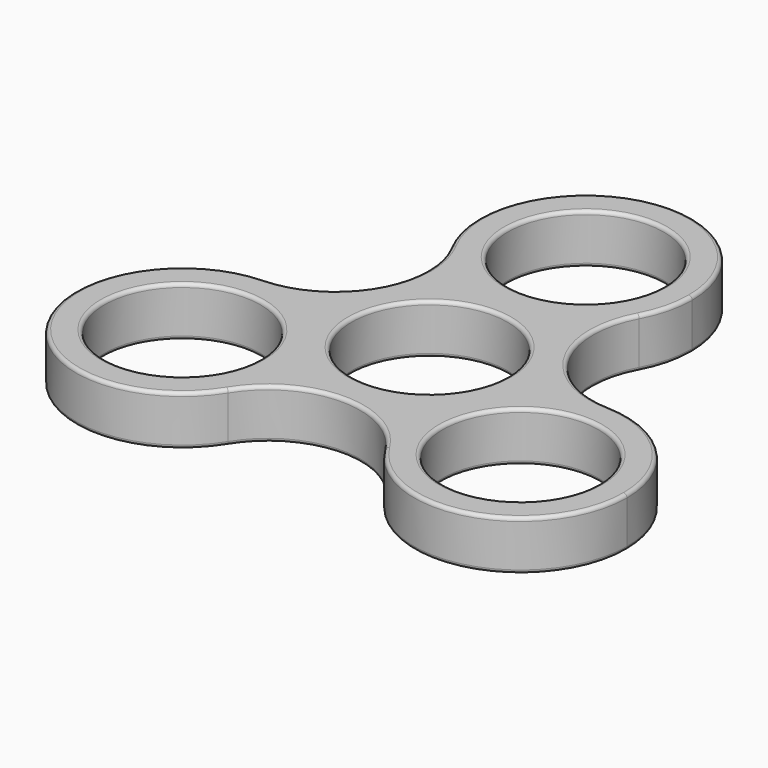
from build123d import *

# Parameters (mm, degrees)
F0_R     = 11
F1_DEPTH = 7
F2_R     = 0.5


# Not quite as in the source:
# - a feature names something its author has since deleted; it is built from what else it names


with BuildPart() as f1:
    # F0 (on Top) → F1 (new body)
    with BuildSketch(Plane.XY):
        with BuildLine():
            ThreePointArc((-61.119560109, 18.0493719403), (-59.7843480604, 21.4909475398), (-59.330106933, 25.1544020325))
            ThreePointArc((-59.330106933, 25.1544020325), (-77.9935614257, 39.7001609051), (-87.540653757, 18.0493719403))
            ThreePointArc((-87.540653757, 18.0493719403), (-84.4913145964, 14.1203701845), (-80.3248963371, 11.4044020325))
            ThreePointArc((-80.3248963371, 11.4044020325), (-74.330106933, 12.6544020325), (-68.3353175289, 11.4044020325))
            ThreePointArc((-68.3353175289, 11.4044020325), (-64.1688992696, 14.1203701845), (-61.119560109, 18.0493719403))
        make_face()
        with Locations((-74.330106933, 25.1544020325)):
            Circle(F0_R, mode=Mode.SUBTRACT)
        with BuildLine():
            ThreePointArc((-80.3248963371, 11.4044020325), (-84.4913145964, 14.1203701845), (-87.540653757, 18.0493719403))
            ThreePointArc((-87.540653757, 18.0493719403), (-87.7314640886, 5.3916791938), (-98.5979423946, -1.102413774))
            ThreePointArc((-98.5979423946, -1.102413774), (-93.6706574823, -1.7787180739), (-89.2353509371, -4.0289580532))
            ThreePointArc((-89.2353509371, -4.0289580532), (-87.3204879898, 5.1544020325), (-80.3248963371, 11.4044020325))
        make_face()
        with BuildLine():
            ThreePointArc((-50.0622714714, -1.102413774), (-60.9287497774, 5.3916791938), (-61.119560109, 18.0493719403))
            ThreePointArc((-61.119560109, 18.0493719403), (-64.1688992696, 14.1203701845), (-68.3353175289, 11.4044020325))
            ThreePointArc((-68.3353175289, 11.4044020325), (-61.7817635949, 5.8726183517), (-59.330106933, -2.3455979675))
            ThreePointArc((-59.330106933, -2.3455979675), (-59.3538146672, -3.1886104047), (-59.4248629289, -4.0289580532))
            ThreePointArc((-59.4248629289, -4.0289580532), (-54.9895563837, -1.7787180739), (-50.0622714714, -1.102413774))
        make_face()
        with BuildLine():
            ThreePointArc((-68.3353175289, 11.4044020325), (-74.330106933, 12.6544020325), (-80.3248963371, 11.4044020325))
            ThreePointArc((-80.3248963371, 11.4044020325), (-74.330106933, 10.1544020325), (-68.3353175289, 11.4044020325))
        make_face()
        with BuildLine():
            ThreePointArc((-68.3353175289, 11.4044020325), (-74.330106933, 10.1544020325), (-80.3248963371, 11.4044020325))
            ThreePointArc((-80.3248963371, 11.4044020325), (-87.3204879898, 5.1544020325), (-89.2353509371, -4.0289580532))
            ThreePointArc((-89.2353509371, -4.0289580532), (-85.1554244803, -8.5955979675), (-83.240561533, -14.4122378818))
            ThreePointArc((-83.240561533, -14.4122378818), (-74.330106933, -17.3455979675), (-65.419652333, -14.4122378818))
            ThreePointArc((-65.419652333, -14.4122378818), (-63.5047893857, -8.5955979675), (-59.4248629289, -4.0289580532))
            ThreePointArc((-59.4248629289, -4.0289580532), (-59.3538146672, -3.1886104047), (-59.330106933, -2.3455979675))
            ThreePointArc((-59.330106933, -2.3455979675), (-61.7817635949, 5.8726183517), (-68.3353175289, 11.4044020325))
        make_face()
        with Locations((-74.330106933, -2.3455979675)):
            Circle(F0_R, mode=Mode.SUBTRACT)
        with BuildLine():
            ThreePointArc((-89.2353509371, -4.0289580532), (-93.6706574823, -1.7787180739), (-98.5979423946, -1.102413774))
            ThreePointArc((-98.5979423946, -1.102413774), (-111.1361865938, -23.5955979675), (-85.3873955706, -23.9837520689))
            ThreePointArc((-85.3873955706, -23.9837520689), (-83.7170815897, -20.1958327476), (-83.1458055371, -16.0955979675))
            ThreePointArc((-83.1458055371, -16.0955979675), (-83.1695132713, -15.2525855304), (-83.240561533, -14.4122378818))
            ThreePointArc((-83.240561533, -14.4122378818), (-87.3204879898, -9.8455979675), (-89.2353509371, -4.0289580532))
        make_face()
        with Locations((-98.1458055371, -16.0955979675)):
            Circle(F0_R, mode=Mode.SUBTRACT)
        with BuildLine():
            ThreePointArc((-35.5144083289, -16.0955979675), (-39.7491388743, -5.650073875), (-50.0622714714, -1.102413774))
            ThreePointArc((-50.0622714714, -1.102413774), (-54.9895563837, -1.7787180739), (-59.4248629289, -4.0289580532))
            ThreePointArc((-59.4248629289, -4.0289580532), (-61.3397258762, -9.8455979675), (-65.419652333, -14.4122378818))
            ThreePointArc((-65.419652333, -14.4122378818), (-65.1507640471, -19.3784460131), (-63.2728182954, -23.9837520689))
            ThreePointArc((-63.2728182954, -23.9837520689), (-46.4141735489, -30.5243219149), (-35.5144083289, -16.0955979675))
        make_face()
        with Locations((-50.5144083289, -16.0955979675)):
            Circle(F0_R, mode=Mode.SUBTRACT)
        with BuildLine():
            ThreePointArc((-83.240561533, -14.4122378818), (-85.1554244803, -8.5955979675), (-89.2353509371, -4.0289580532))
            ThreePointArc((-89.2353509371, -4.0289580532), (-87.3204879898, -9.8455979675), (-83.240561533, -14.4122378818))
        make_face()
        with BuildLine():
            ThreePointArc((-83.1458055371, -16.0955979675), (-83.7170815897, -20.1958327476), (-85.3873955706, -23.9837520689))
            ThreePointArc((-85.3873955706, -23.9837520689), (-74.330106933, -17.8201522901), (-63.2728182954, -23.9837520689))
            ThreePointArc((-63.2728182954, -23.9837520689), (-65.1507640471, -19.3784460131), (-65.419652333, -14.4122378818))
            ThreePointArc((-65.419652333, -14.4122378818), (-74.330106933, -17.3455979675), (-83.240561533, -14.4122378818))
            ThreePointArc((-83.240561533, -14.4122378818), (-83.1695132713, -15.2525855304), (-83.1458055371, -16.0955979675))
        make_face()
        with BuildLine():
            ThreePointArc((-65.419652333, -14.4122378818), (-61.3397258762, -9.8455979675), (-59.4248629289, -4.0289580532))
            ThreePointArc((-59.4248629289, -4.0289580532), (-63.5047893857, -8.5955979675), (-65.419652333, -14.4122378818))
        make_face()
    extrude(amount=F1_DEPTH)

    # F2
    f2_edges = [f1.edges().sort_by_distance(p)[0] for p in [
        (-111.136187, -23.595598, 0),
        (-74.330107, -17.820152, 0),
        (-37.524027, -23.595598, 0),
        (-60.92875, 5.391679, 0),
        (-74.330107, 40.154402, 0),
        (-87.731464, 5.391679, 0),
        (-109.145806, -16.095598, 0),
        (-61.514408, -16.095598, 0),
        (-85.330107, -2.345598, 0),
        (-85.330107, 25.154402, 0),
        (-111.136187, -23.595598, 7),
        (-74.330107, -17.820152, 7),
        (-37.524027, -23.595598, 7),
        (-60.92875, 5.391679, 7),
        (-74.330107, 40.154402, 7),
        (-87.731464, 5.391679, 7),
        (-109.145806, -16.095598, 7),
        (-61.514408, -16.095598, 7),
        (-85.330107, -2.345598, 7),
        (-85.330107, 25.154402, 7),
    ]]
    fillet(f2_edges, radius=F2_R)


solid = f1.part
